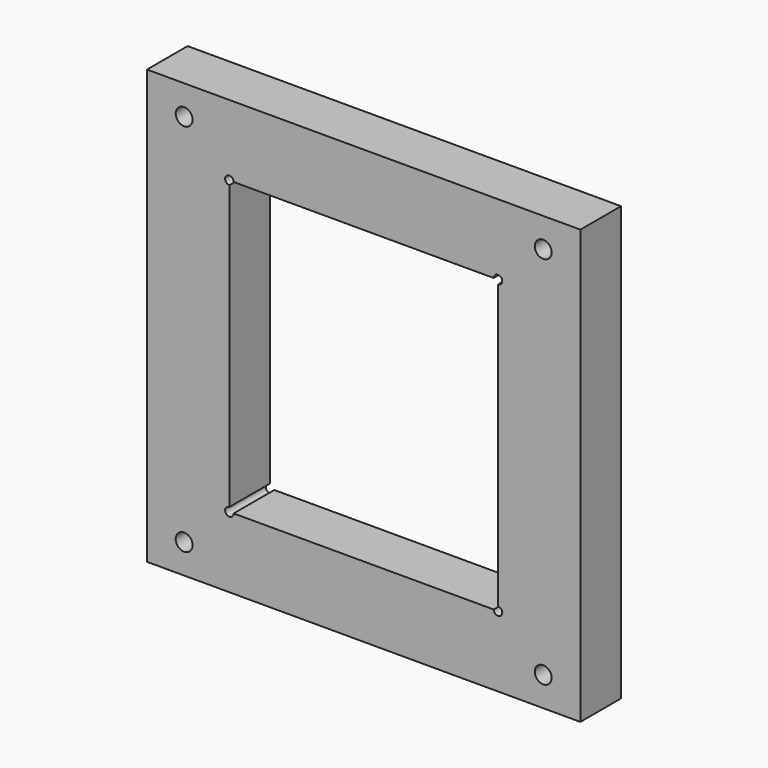
from build123d import *

# Parameters (mm, degrees)
F0_W     = 81.28
F0_H     = 81.28
F0_W_2   = 50.377
F0_H_2   = 54.727
F1_DEPTH = 9.525
F3_D     = 3.175
F4_D     = 1.6002


# Not quite as in the source:
# - a feature names something its author has since deleted; it is built from what else it names


with BuildPart() as f1:
    # F0 (on Front) → F1 (new body)
    with BuildSketch(Plane.XZ):
        Rectangle(F0_W, F0_H)
        Rectangle(F0_W_2, F0_H_2, mode=Mode.SUBTRACT)
    extrude(amount=F1_DEPTH)

    # F3 (through all)
    with Locations(Plane.XZ.offset(9.525)):
        with Locations((-33.6692971992, 35.1226272138), (33.6692971992, 35.1226272138), (-33.6692971992, -35.1226272138), (33.6692971992, -35.1226272138)):
            Hole(F3_D / 2)

    # F4 (through all)
    with Locations(Plane(origin=(0, 0, 0), x_dir=(1, 0, 0), z_dir=(0, 1, 0))):
        with Locations((25.1885, -27.3635), (-25.1885, -27.3635), (-25.1885, 27.3635), (25.1885, 27.3635)):
            Hole(F4_D / 2)


solid = f1.part
